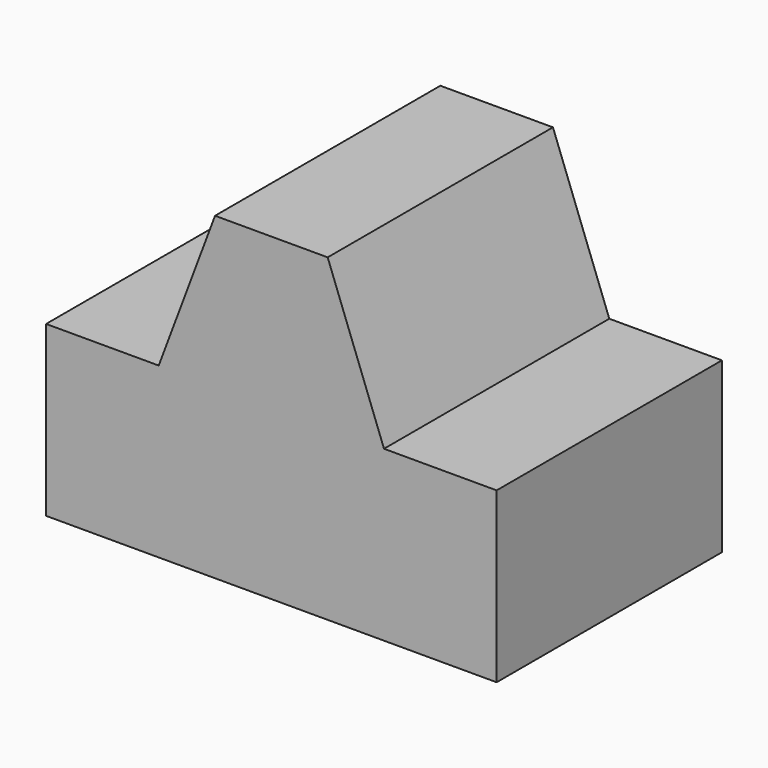
from build123d import *

# Parameters (mm, degrees)
F1_DEPTH = 750


# Not quite as in the source:
# - a pattern or mirror of a feature is missing from the dataset's text; its kind, count and spacing are read off the source's solid


with BuildPart() as f1:
    # F0 (on Front) → F1 (new body)
    with BuildSketch(Plane.XZ):
        Polygon((0, 450), (0, 0), (600, 0), (600, 450), (300, 450), align=None)
        Polygon((0, 850), (0, 450), (300, 450), (150, 850), align=None)
    extrude(amount=F1_DEPTH)

    # F1_copies: F1 across plane


with BuildPart() as f1_1:
    add(f1.part)
    add(f1.part.mirror(Plane(origin=(0, 0, 0), x_dir=(0, 0, -1), z_dir=(-1, 0, 0))))


solid = f1_1.part
